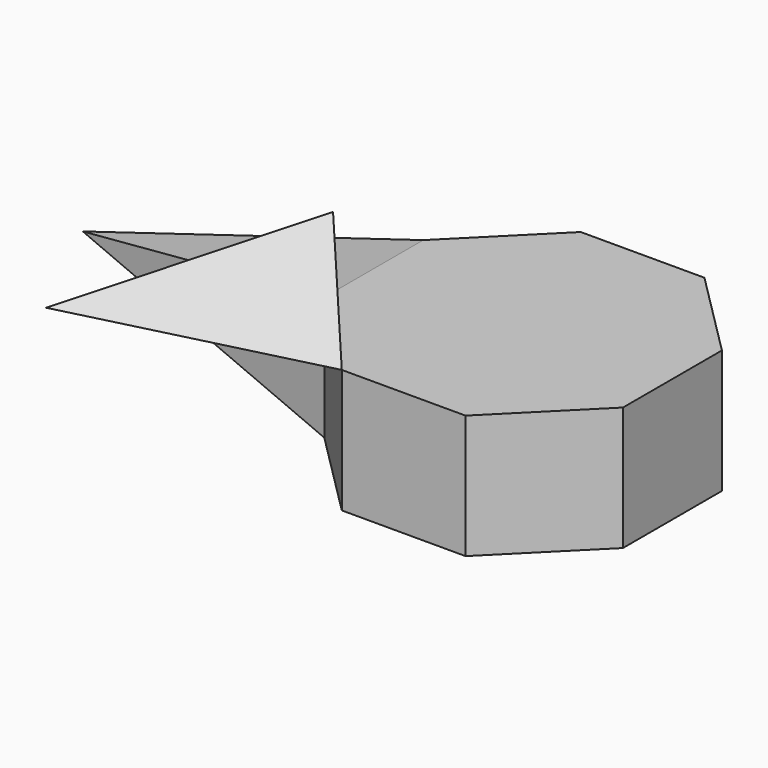
from build123d import *

# Parameters (mm, degrees)
F1_DEPTH  = 25
F1_FACE_W = 25
F1_FACE_H = 25


# Not quite as in the source:
# - an extrude whose draft closes it to a point is written as a loft to that point


with BuildPart() as f1:
    # F0 (on Top) → F1 (new body)
    with BuildSketch(Plane.XY):
        Polygon((12.5, -30.1776695297), (30.1776695297, -12.5), (30.1776695297, 12.5), (12.5, 30.1776695297), (-12.5, 30.1776695297), (-30.1776695297, 12.5), (-30.1776695297, -12.5), (-12.5, -30.1776695297), align=None)
    extrude(amount=F1_DEPTH)


with BuildPart() as f2:
    # F1_face (on face) → F2 section 0
    with BuildSketch(Plane(origin=(-30.1776695297, 0, 12.5), x_dir=(0, -1, 0), z_dir=(-1, 0, 0)), mode=Mode.PRIVATE) as f2_s0:
        Rectangle(F1_FACE_W, F1_FACE_H)
    loft([f2_s0.sketch, Vertex(-88.9855458981, 0, 12.5)], ruled=True)


with BuildPart() as f4:
    # F3 (on face) → F4 section 0
    with BuildSketch(Plane(origin=(-21.3388347648, -21.3388347648, 0), x_dir=(0.7071067812, -0.7071067812, 0), z_dir=(-0.7071067812, -0.7071067812, 0)), mode=Mode.PRIVATE) as f4_s0:
        Polygon((-12.5, 25), (12.5, 25), (0, 46.6506350946), align=None)
    loft([f4_s0.sketch, Vertex(-53.5585630433, -53.5585630433, 32.2168783649)], ruled=True)


solid = Compound([f1.part, f2.part, f4.part])
